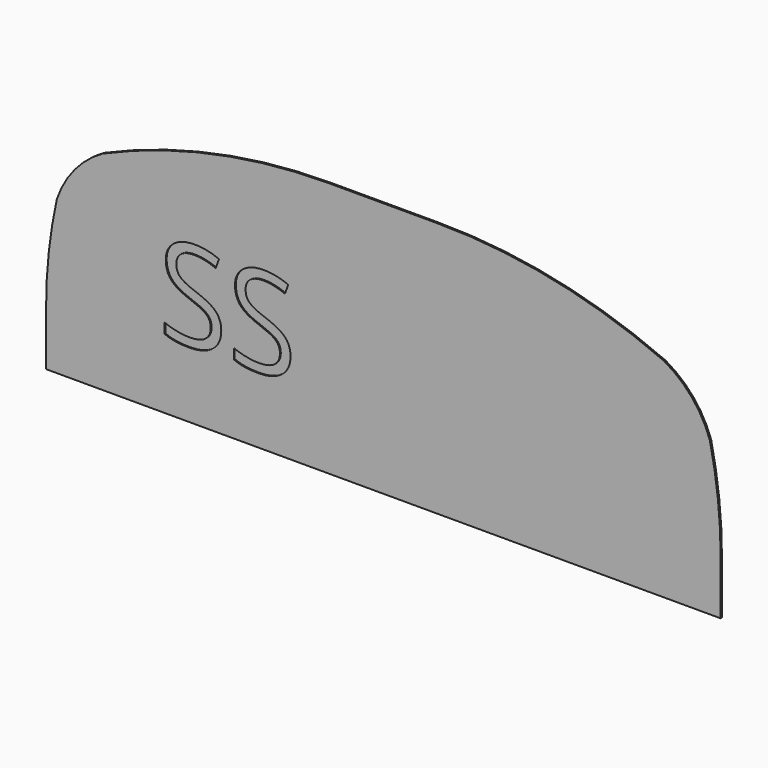
from build123d import *

# Parameters (mm, degrees)
F1_DEPTH     = 3
F2_TEXT_SIZE = 231.8762242794
F3_DEPTH     = 2


# Not quite as in the source:
# - Text() gives the source's letters only with a copy of the font that has no kerning and outlines rounded to 1/6400 em; it was checked with that copy


with BuildPart() as f1:
    # F0 (on Front) → F1 (new body)
    with BuildSketch(Plane.XZ):
        with BuildLine():
            Line((-620, 0), (0, 0))
            Line((0, 0), (620, 0))
            Line((620, 0), (620, 100))
            ThreePointArc((620, 100), (615.0412777663, 191.3677432028), (600.2233624458, 281.6621661186))
            ThreePointArc((600.2233624458, 281.6621661186), (567.5601803208, 339.9425725873), (516.1690115929, 382.6325833797))
            ThreePointArc((516.1690115929, 382.6325833797), (312.6203845455, 447.9226553518), (100, 470))
            Line((100, 470), (0, 470))
            Line((0, 470), (-100, 470))
            ThreePointArc((-100, 470), (-312.6203845455, 447.9226553518), (-516.1690115929, 382.6325833797))
            ThreePointArc((-516.1690115929, 382.6325833797), (-567.5601803208, 339.9425725873), (-600.2233624458, 281.6621661186))
            ThreePointArc((-600.2233624458, 281.6621661186), (-615.0412777663, 191.3677432028), (-620, 100))
            Line((-620, 100), (-620, 0))
        make_face()
    extrude(amount=F1_DEPTH)

    # F2 (on face) → F3 (cut)
    with BuildSketch(Plane.XZ.offset(3)):
        with Locations((-414.1249209642, 122.6973384619)):
            Text('SS', F2_TEXT_SIZE, font='Open Sans', text_align=(TextAlign.LEFT, TextAlign.BOTTOM))
    extrude(amount=-F3_DEPTH, mode=Mode.SUBTRACT)


solid = f1.part
